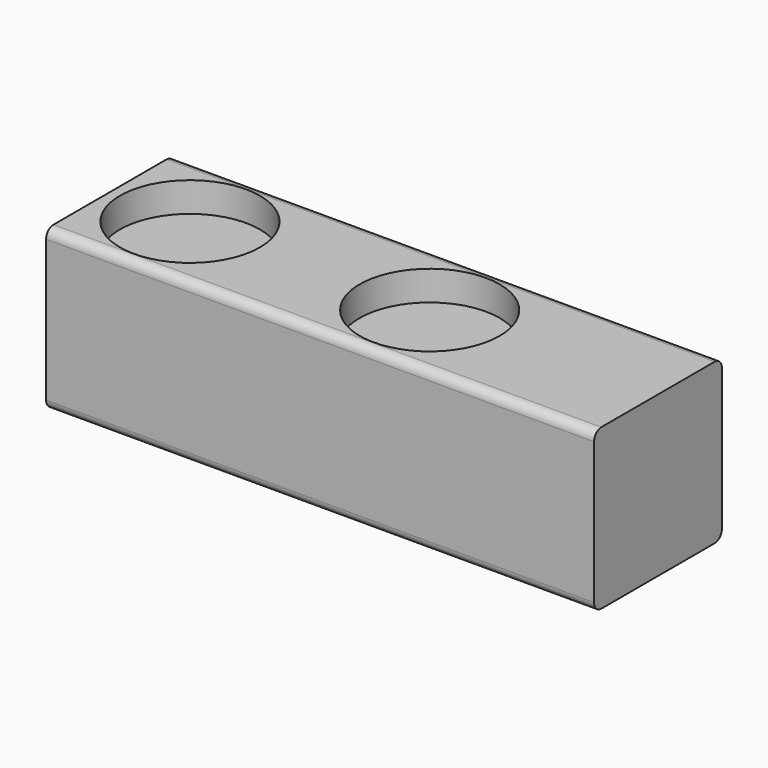
from build123d import *

# Parameters (mm, degrees)
F0_W          = 88.9
F0_H          = 88.9
F1_DEPTH      = 152.4
F1_DEPTH_BACK = 152.4
F2_R          = 38.9255
F3_DEPTH      = 16.51
F4_R          = 5.08


with BuildPart() as f1:
    # F0 (on Right) → F1 (new body, two sides)
    with BuildSketch(Plane.YZ) as f1_sk:
        Rectangle(F0_W, F0_H)
    extrude(amount=F1_DEPTH)
    extrude(f1_sk.sketch, amount=-F1_DEPTH_BACK)

    # F2 (on face) → F3 (cut)
    with BuildSketch(Plane.XY.offset(44.45)):
        with Locations((-107.95, 0)):
            Circle(F2_R)
        with Locations((25.4, 0)):
            Circle(F2_R)
    extrude(amount=-F3_DEPTH, mode=Mode.SUBTRACT)

    # F4
    f4_edges = [f1.edges().sort_by_distance(p)[0] for p in [
        (0, -44.45, 44.45),
        (0, 44.45, 44.45),
        (0, -44.45, -44.45),
        (0, 44.45, -44.45),
    ]]
    fillet(f4_edges, radius=F4_R)


solid = f1.part
